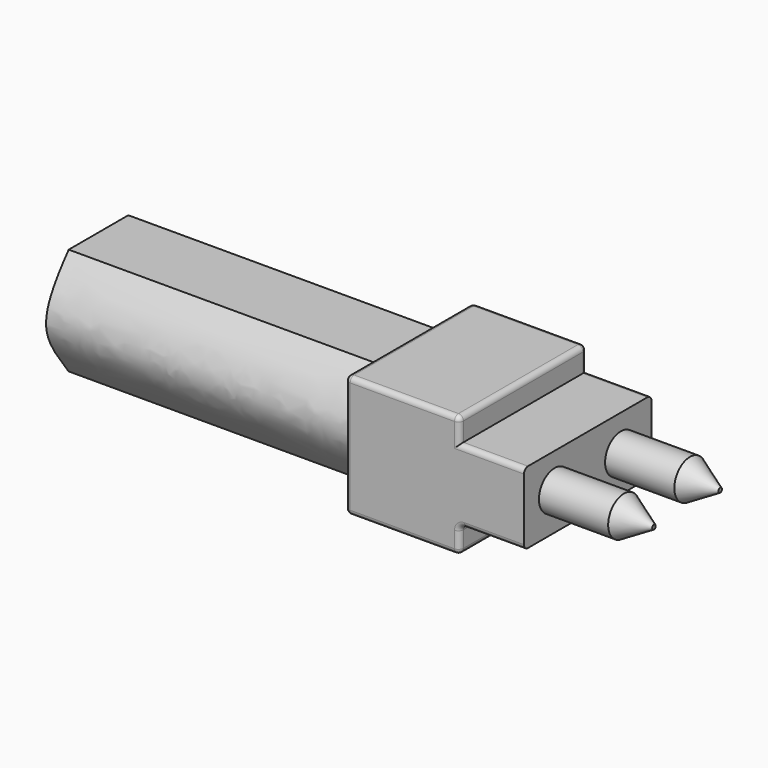
from build123d import *

# Parameters (mm, degrees)
F1_W       = 7.2
F1_H       = 6.41
F2_DEPTH   = 2.9
F3_W       = 4.6
F3_H       = 6.41
F4_DEPTH   = 0.955
F5_DEPTH   = 3.955
F6_R       = 0.2
F7_R       = 0.79
F8_DEPTH   = 4
F9_SIZE2   = 0.7
F9_SIZE    = 1.2124355653
F9_2_SIZE2 = 0.7
F9_2_SIZE  = 1.2124355653
F11_DEPTH  = 12.5


# Not quite as in the source:
# - a feature names something its author has since deleted; it is built from what else it names


with BuildPart() as f2:
    # F1 (on face) → F2 (new body)
    with BuildSketch(Plane.XY):
        with Locations((1.1224337457, -1.1278976017)):
            Rectangle(F1_W, F1_H)
    extrude(amount=F2_DEPTH)

    # F3 (on face) → F4 (join)
    with BuildSketch(Plane.XY.offset(2.9)):
        with Locations((-0.1775662543, -1.1278976017)):
            Rectangle(F3_W, F3_H)
    extrude(amount=F4_DEPTH)

    # F3 (on face) → F5 (join)
    with BuildSketch(Plane.XY.offset(2.9)):
        with Locations((-0.1775662543, -1.1278976017)):
            Rectangle(F3_W, F3_H)
    extrude(amount=-F5_DEPTH)

    # F6
    f6_edges = [f2.edges().sort_by_distance(p)[0] for p in [
        (2.122434, -1.127898, 3.855),
        (-0.177566, -4.332898, 3.855),
        (-2.477566, -1.127898, 3.855),
        (-0.177566, 2.077102, 3.855),
        (3.422434, -4.332898, 2.9),
        (2.122434, -4.332898, 3.3775),
        (-2.477566, -4.332898, 1.4),
        (-0.177566, -4.332898, -1.055),
        (2.122434, -1.127898, -1.055),
        (-0.177566, 2.077102, -1.055),
        (2.122434, -4.332898, -0.5275),
        (3.422434, -4.332898, 0),
        (2.122434, 2.077102, -0.5275),
        (3.422434, 2.077102, 2.9),
        (2.122434, 2.077102, 3.3775),
        (3.422434, 2.077102, 0),
        (-2.477566, 2.077102, 1.4),
        (-2.477566, -1.127898, -1.055),
        (2.122434, -1.127898, 0),
    ]]
    fillet(f6_edges, radius=F6_R)

    # F7 (on face) → F8 (join)
    with BuildSketch(Plane.YZ.offset(4.7224337457)):
        with Locations((-2.7930222052, 1.5)):
            Circle(F7_R)
        with Locations((0.5366023983, 1.45)):
            Circle(F7_R)
    extrude(amount=F8_DEPTH)

    # F9
    f9_edges = [f2.edges().sort_by_distance(p)[0] for p in [
        (8.722434, -3.583022, 1.5),
    ]]
    f9_side = f2.faces().sort_by_distance((6.722434, -3.583022, 1.5))[0]
    chamfer(f9_edges, length=F9_SIZE, length2=F9_SIZE2, reference=f9_side)

    # F9#2
    f9_2_edges = [f2.edges().sort_by_distance(p)[0] for p in [
        (8.722434, -0.253398, 1.45),
    ]]
    f9_2_side = f2.faces().sort_by_distance((6.722434, -0.253398, 1.45))[0]
    chamfer(f9_2_edges, length=F9_2_SIZE, length2=F9_2_SIZE2, reference=f9_2_side)

    # F10 (on face) → F11 (join)
    with BuildSketch(Plane(origin=(-2.4775662543, 0, 0), x_dir=(0, -1, 0), z_dir=(-1, 0, 0))):
        with BuildLine():
            Line((2.6228976017, 3.555), (-0.3771023983, 3.555))
            add(Edge.make_bspline(
                [(-0.3771023983, 3.555), (-0.9371962785, 2.8481079618), (-2.0580811679, 1.3923591855), (-0.9290927555, -0.0252525917), (-0.3671023983, -0.755)],
                knots=[0, 0, 0, 0, 0.4994437063, 1, 1, 1, 1], degree=3))
            Line((-0.3671023983, -0.755), (2.6328976017, -0.755))
            add(Edge.make_bspline(
                [(2.6328976017, -0.755), (3.1901916784, 0.0098145578), (4.3309296415, 1.3596346202), (3.1935954585, 2.8839832867), (2.6228976017, 3.555)],
                knots=[0, 0, 0, 0, 0.5000783208, 1, 1, 1, 1], degree=3))
        make_face()
    extrude(amount=F11_DEPTH)


solid = f2.part
